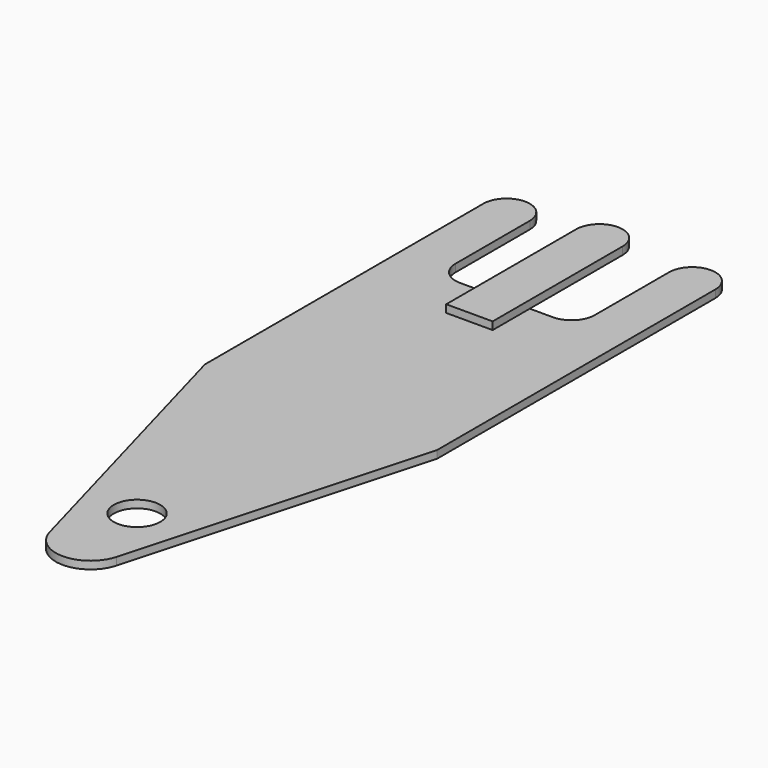
from build123d import *

# Parameters (mm, degrees)
F1_DEPTH    = 1.05
F2_R        = 3.175
F3_DEPTH    = 28.1652770936
F4_T1_DEPTH = 16.925
F6_DEPTH    = 1.05
F7_DEPTH    = 6.35
F8_DEPTH    = 1.05
F9_R        = 3.175


# Not quite as in the source:
# - a fillet or chamfer that OpenCascade refuses, or shapes differently, is made with other operations: its cross-section is extruded or revolved along the edge and cut away or added


with BuildPart() as f1:
    # F0 (on Top) → F1 (new body)
    with BuildSketch(Plane.XY):
        Polygon((-15.875, 0), (15.875, 0), (15.875, 50.8), (9.525, 50.8), (9.525, 31.75), (3.175, 31.75), (3.175, 50.8), (-3.175, 50.8), (-3.175, 31.75), (-9.525, 31.75), (-9.525, 50.8), (-15.875, 50.8), align=None)
        with BuildLine():
            Line((4.5889374784, -40.6525160217), (15.875, 0))
            Line((15.875, 0), (-15.875, 0))
            Line((-15.875, 0), (-4.5889374784, -40.6525160217))
            ThreePointArc((-4.5889374784, -40.6525160217), (0, -44.1410226664), (4.5889374784, -40.6525160217))
        make_face()
    extrude(amount=F1_DEPTH)

    # F2 (on face) → F3 (cut)
    with BuildSketch(Plane.XY):
        with Locations((0, -31.4410226664)):
            Circle(F2_R)
    extrude(amount=F3_DEPTH, mode=Mode.SUBTRACT)

    # F4: fillet of radius 3.175 on 6 edges, made by hand

    # F4_s2 → F4_t1 (cut)
    with BuildSketch(Plane.XY.offset(-7.9375)):
        with BuildLine():
            ThreePointArc((15.875, 47.625), (14.9450640303, 49.8700640303), (12.7, 50.8))
            Line((12.7, 50.8), (15.875, 50.8))
            Line((15.875, 50.8), (15.875, 47.625))
        make_face()
        with BuildLine():
            ThreePointArc((12.7, 50.8), (10.4549359697, 49.8700640303), (9.525, 47.625))
            Line((9.525, 47.625), (9.525, 50.8))
            Line((9.525, 50.8), (12.7, 50.8))
        make_face()
        with BuildLine():
            ThreePointArc((3.175, 47.625), (2.2450640303, 49.8700640303), (0, 50.8))
            Line((0, 50.8), (3.175, 50.8))
            Line((3.175, 50.8), (3.175, 47.625))
        make_face()
        with BuildLine():
            ThreePointArc((0, 50.8), (-2.2450640303, 49.8700640303), (-3.175, 47.625))
            Line((-3.175, 47.625), (-3.175, 50.8))
            Line((-3.175, 50.8), (0, 50.8))
        make_face()
        with BuildLine():
            ThreePointArc((-12.7, 50.8), (-10.4549359697, 49.8700640303), (-9.525, 47.625))
            Line((-9.525, 47.625), (-9.525, 50.8))
            Line((-9.525, 50.8), (-12.7, 50.8))
        make_face()
        with BuildLine():
            ThreePointArc((-15.875, 47.625), (-14.9450640303, 49.8700640303), (-12.7, 50.8))
            Line((-12.7, 50.8), (-15.875, 50.8))
            Line((-15.875, 50.8), (-15.875, 47.625))
        make_face()
    extrude(amount=F4_T1_DEPTH, mode=Mode.SUBTRACT)

    # F5 (on face) → F6 (join)
    with BuildSketch(Plane.XY.offset(1.05)):
        with BuildLine():
            Line((-3.175, 47.625), (-3.175, 31.75))
            Line((-3.175, 31.75), (3.175, 31.75))
            Line((3.175, 31.75), (3.175, 47.625))
            ThreePointArc((3.175, 47.625), (0, 50.8), (-3.175, 47.625))
        make_face()
    extrude(amount=F6_DEPTH)

    # F7 (add): a face of the model
    f7_faces = [f1.faces().sort_by_distance(p)[0] for p in [
        (0, 31.75, 1.575),
    ]]
    extrude(f7_faces, amount=F7_DEPTH)

    # F5 (on face) → F8 (cut)
    with BuildSketch(Plane.XY.offset(1.05)):
        with BuildLine():
            Line((-3.175, 47.625), (-3.175, 31.75))
            Line((-3.175, 31.75), (3.175, 31.75))
            Line((3.175, 31.75), (3.175, 47.625))
            ThreePointArc((3.175, 47.625), (0, 50.8), (-3.175, 47.625))
        make_face()
    extrude(amount=-F8_DEPTH, mode=Mode.SUBTRACT)

    # F9
    f9_edges = [f1.edges().sort_by_distance(p)[0] for p in [
        (-9.525, 31.75, 0.525),
        (9.525, 31.75, 0.525),
    ]]
    fillet(f9_edges, radius=F9_R)


solid = f1.part
